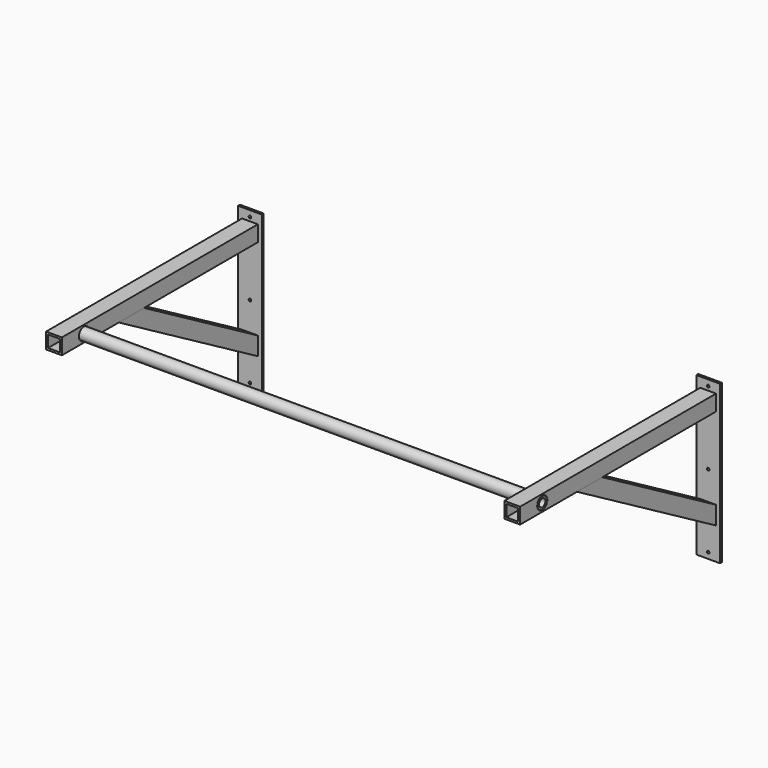
from build123d import *

# Parameters (mm, degrees)
F0_R          = 15
F0_R_2        = 10
F1_DEPTH      = 600
F1_DEPTH_BACK = 600
F3_W          = 40
F3_H          = 40
F3_W_2        = 30
F3_H_2        = 30
F4_DEPTH      = 620
F5_R          = 16
F6_DEPTH      = 53.9
F7_W          = 60
F7_H          = 400
F7_R          = 3.25
F8_DEPTH      = 6
F10_W         = 40
F10_H         = 40
F10_W_2       = 30
F10_H_2       = 30
F11_FACE_W    = 40
F11_FACE_H    = 40
F11_FACE_W_2  = 30
F11_FACE_H_2  = 30
F12_REACH     = 626.0052928413


with BuildPart() as f1:
    # F0 (on Right) → F1 (new body, two sides)
    with BuildSketch(Plane.YZ) as f1_sk:
        Circle(F0_R)
        Circle(F0_R_2, mode=Mode.SUBTRACT)
    extrude(amount=F1_DEPTH)
    extrude(f1_sk.sketch, amount=-F1_DEPTH_BACK)


with BuildPart() as f4:
    # F3 (on offset) → F4 (new body)
    with BuildSketch(Plane.XZ.offset(-550)):
        with Locations((-580, 0)):
            Rectangle(F3_W, F3_H)
        with Locations((-580, 0)):
            Rectangle(F3_W_2, F3_H_2, mode=Mode.SUBTRACT)
    extrude(amount=F4_DEPTH)

    # F5 (on face) → F6 (cut)
    with BuildSketch(Plane(origin=(-600, 0, 0), x_dir=(0, -1, 0), z_dir=(-1, 0, 0))):
        Circle(F5_R)
    extrude(amount=-F6_DEPTH, mode=Mode.SUBTRACT)


with BuildPart() as f8:
    # F7 (on offset) → F8 (new body)
    with BuildSketch(Plane.XZ.offset(-550)):
        with Locations((-580, -155)):
            Rectangle(F7_W, F7_H)
        with Locations((-580, -340)):
            Circle(F7_R, mode=Mode.SUBTRACT)
        with Locations((-580, -155)):
            Circle(F7_R, mode=Mode.SUBTRACT)
        with Locations((-580, 30)):
            Circle(F7_R, mode=Mode.SUBTRACT)
    extrude(amount=-F8_DEPTH)


with BuildPart() as f11:
    # F10 (on face) → F11 (new body, up to the next surface of F8)
    with BuildSketch(Plane(origin=(0, 421.1602540378, -243.1569860407), x_dir=(-1, 0, 0), z_dir=(0, 0.8660254038, -0.5))):
        with Locations((580, 57.6794919243)):
            Rectangle(F10_W, F10_H)
        with Locations((580, 57.6794919243)):
            Rectangle(F10_W_2, F10_H_2, mode=Mode.SUBTRACT)
    extrude(until=Until.NEXT, target=f8.part)

    f12_end = f4.part.faces().sort_by_distance((-580, 240, -20))[0]
    # F11_face (on face) → F12 (join, up to a face of F4 that its end follows)
    with BuildSketch(Plane(origin=(-580, 450, -193.2050807569), x_dir=(-1, 0, 0), z_dir=(0, -0.8660254038, 0.5))):
        Rectangle(F11_FACE_W, F11_FACE_H)
        Rectangle(F11_FACE_W_2, F11_FACE_H_2, mode=Mode.SUBTRACT)
    f12_long = extrude(amount=F12_REACH, mode=Mode.PRIVATE)
    add(split(f12_long, bisect_by=f12_end, keep=Keep.TOP, mode=Mode.PRIVATE))


with BuildPart() as f13_1:
    # F13: instance of F4
    add(f4.part.mirror(Plane.YZ))


with BuildPart() as f13_2:
    # F13: instance of F8
    add(f8.part.mirror(Plane.YZ))


with BuildPart() as f13_3:
    # F13: instance of F11
    add(f11.part.mirror(Plane.YZ))


solid = Compound([f1.part, f4.part, f8.part, f11.part, f13_1.part, f13_2.part, f13_3.part])
